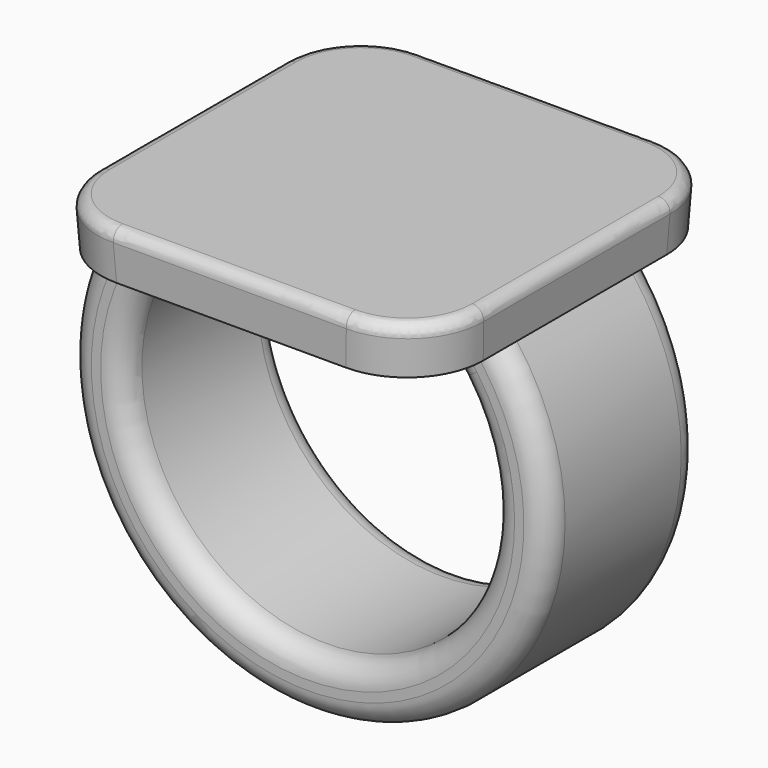
from build123d import *

# Parameters (mm, degrees)
F0_W          = 25.4
F0_H          = 25.4
F1_DEPTH      = 3.175
F1_TAPER      = -3
F3_W          = 5.08
F3_H          = 12.7
F6_DEPTH      = 6.35
F6_DEPTH_BACK = 6.35
F7_R          = 5.08
F8_R          = 1.524
F9_R          = 0.762


with BuildPart() as f1:
    # F0 (on Top) → F1 (new body)
    with BuildSketch(Plane.XY):
        Rectangle(F0_W, F0_H)
    extrude(amount=F1_DEPTH, taper=F1_TAPER)

    # F4: sweep along a path in F2
    with BuildLine(Plane.XZ) as f4_path:
        ThreePointArc((-10.16, 0), (0, -23.5582897328), (10.16, 0))
    # F3 (on face) → F4 (sweep)
    with BuildSketch(Plane(origin=(0, 0, 0), x_dir=(1, 0, 0), z_dir=(0, 0, -1))):
        with Locations((-10.16, 0)):
            Rectangle(F3_W, F3_H)
    sweep(path=f4_path.line)

    # F5 (on Front) → F6 (join, two sides)
    with BuildSketch(Plane.XZ) as f6_sk:
        with BuildLine():
            Line((10.16, 0), (7.62, 0))
            ThreePointArc((7.62, 0), (8.9072265211, -1.1822790439), (10.0130578512, -2.535746045))
            Line((10.0130578512, -2.535746045), (10.16, 0))
        make_face()
    extrude(amount=F6_DEPTH)
    extrude(f6_sk.sketch, amount=-F6_DEPTH_BACK)

    # F7
    f7_edges = [f1.edges().sort_by_distance(p)[0] for p in [
        (-12.783197, -12.783197, 1.5875),
        (-12.783197, 12.783197, 1.5875),
        (12.783197, 12.783197, 1.5875),
        (12.783197, -12.783197, 1.5875),
    ]]
    fillet(f7_edges, radius=F7_R)

    # F8
    f8_edges = [f1.edges().sort_by_distance(p)[0] for p in [
        (-1.743325, -6.35, -21.711017),
        (-1.743325, 6.35, -21.711017),
        (8.907227, 6.35, -1.182279),
        (0, 6.35, -25.501344),
        (8.907227, -6.35, -1.182279),
        (0, -6.35, -25.501344),
    ]]
    fillet(f8_edges, radius=F8_R)

    # F9
    f9_edges = [f1.edges().sort_by_distance(p)[0] for p in [
        (0, 12.866395, 3.175),
        (11.381378, 11.381378, 3.175),
        (-11.381378, 11.381378, 3.175),
        (12.866395, 0, 3.175),
        (-12.866395, 0, 3.175),
        (11.381378, -11.381378, 3.175),
        (-11.381378, -11.381378, 3.175),
        (0, -12.866395, 3.175),
    ]]
    fillet(f9_edges, radius=F9_R)


solid = f1.part
